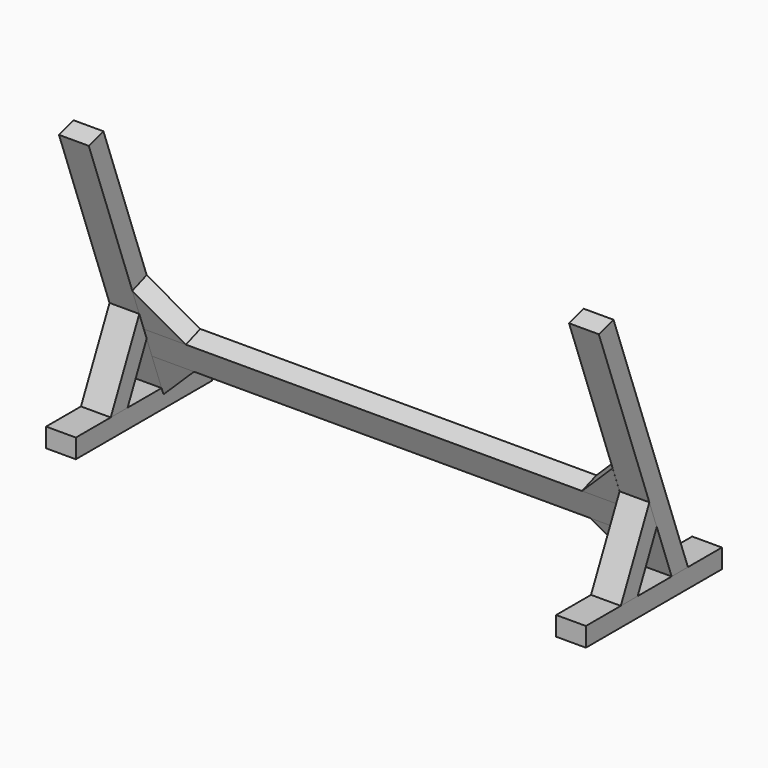
from build123d import *

# Parameters (mm, degrees)
F1_DEPTH = 70
F2_DEPTH = 70
F3_DEPTH = 70
F7_DEPTH = 45
F8_DEPTH = 45


# Not quite as in the source:
# - a feature names something its author has since deleted; it is built from what else it names


with BuildPart() as f1:
    # F0 (on Right) → F1 (new body)
    with BuildSketch(Plane.YZ):
        Polygon((-400, 0), (0, 0), (0, 45), (-100, 45), (-147.782382899, 45), (-247.782382899, 45), (-297.4343892523, 45), (-400, 45), align=None)
    extrude(amount=F1_DEPTH)


with BuildPart() as f2:
    # F0 (on Right) → F2 (new body)
    with BuildSketch(Plane.YZ):
        Polygon((-213.3855698657, 225.2432748353), (-297.4343892523, 45), (-247.782382899, 45), (-191.6195412274, 165.4416026403), align=None)
    extrude(amount=F2_DEPTH)


with BuildPart() as f3:
    # F0 (on Right) → F3 (new body)
    with BuildSketch(Plane.YZ):
        Polygon((-147.782382899, 45), (-100, 45), (-318.8928917284, 646.403277303), (-362.1074258631, 633.8532159676), (-213.3855698657, 225.2432748353), (-191.6195412274, 165.4416026403), align=None)
    extrude(amount=F3_DEPTH)


with BuildPart() as f4_1:
    # F4: instance of F1
    add(f1.part.mirror(Plane.YZ))


with BuildPart() as f4_2:
    # F4: instance of F2
    add(f2.part.mirror(Plane.YZ))


with BuildPart() as f4_3:
    # F4: instance of F3
    add(f3.part.mirror(Plane.YZ))


with BuildPart() as f4_1_1:
    # F5: moved
    add(f4_1.part.moved(Location((-1130, 0, 0))))


with BuildPart() as f4_2_1:
    # F5: moved
    add(f4_2.part.moved(Location((-1130, 0, 0))))


with BuildPart() as f4_3_1:
    # F5: moved
    add(f4_3.part.moved(Location((-1130, 0, 0))))


with BuildPart() as f7:
    # F6 (on face) → F7 (new body)
    with BuildSketch(Plane(origin=(0, -73.839500938, -26.8753804545), x_dir=(-1, 0, 0), z_dir=(0, 0.9396926208, 0.3420201433))):
        Polygon((98.9949493661, 245.483131634), (0, 245.483131634), (0, 175.483131634), (98.9949493661, 175.483131634), (1031.0050506339, 175.483131634), (1130, 175.483131634), (1130, 245.483131634), (1031.0050506339, 245.483131634), align=None)
    extrude(amount=-F7_DEPTH)


with BuildPart() as f8:
    # F6 (on face) → F8 (new body)
    with BuildSketch(Plane(origin=(0, -73.839500938, -26.8753804545), x_dir=(-1, 0, 0), z_dir=(0, 0.9396926208, 0.3420201433))):
        Polygon((0, 344.4780810002), (0, 245.483131634), (98.9949493661, 245.483131634), align=None)
    extrude(amount=-F8_DEPTH)


with BuildPart() as f8b:
    # F6 (on face) → F8, piece 2 (new body)
    with BuildSketch(Plane(origin=(0, -73.839500938, -26.8753804545), x_dir=(-1, 0, 0), z_dir=(0, 0.9396926208, 0.3420201433))):
        Polygon((98.9949493661, 175.483131634), (0, 175.483131634), (0, 76.4881822679), align=None)
    extrude(amount=-F8_DEPTH)


with BuildPart() as f8c:
    # F6 (on face) → F8, piece 3 (new body)
    with BuildSketch(Plane(origin=(0, -73.839500938, -26.8753804545), x_dir=(-1, 0, 0), z_dir=(0, 0.9396926208, 0.3420201433))):
        Polygon((1130, 175.483131634), (1031.0050506339, 175.483131634), (1130, 76.4881822679), align=None)
    extrude(amount=-F8_DEPTH)


with BuildPart() as f8d:
    # F6 (on face) → F8, piece 4 (new body)
    with BuildSketch(Plane(origin=(0, -73.839500938, -26.8753804545), x_dir=(-1, 0, 0), z_dir=(0, 0.9396926208, 0.3420201433))):
        Polygon((1130, 344.4780810002), (1031.0050506339, 245.483131634), (1130, 245.483131634), align=None)
    extrude(amount=-F8_DEPTH)


solid = Compound([f1.part, f2.part, f3.part, f4_1_1.part, f4_2_1.part, f4_3_1.part, f7.part, f8.part, f8b.part, f8c.part, f8d.part])
